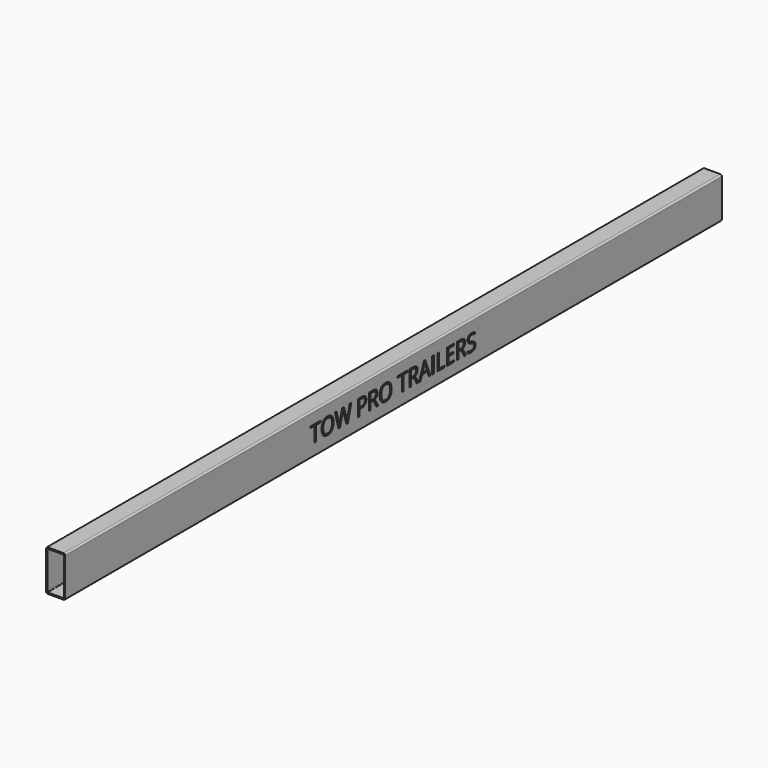
from build123d import *

# Parameters (mm, degrees)
F1_DEPTH      = 1500
F2_TEXT_SIZE  = 41.6666666667
F3_DEPTH      = 25
F3_DEPTH_BACK = 25


# Not quite as in the source:
# - Text() gives the source's letters only with a copy of the font that has no kerning and outlines rounded to 1/6400 em; it was checked with that copy


with BuildPart() as f1:
    # F0 (on Front) → F1 (new body)
    with BuildSketch(Plane.XZ):
        with BuildLine():
            ThreePointArc((17.5, 34.5), (16.6213203436, 36.6213203436), (14.5, 37.5))
            Line((14.5, 37.5), (-14.5, 37.5))
            ThreePointArc((-14.5, 37.5), (-16.6213203436, 36.6213203436), (-17.5, 34.5))
            Line((-17.5, 34.5), (-17.5, -34.5))
            ThreePointArc((-17.5, -34.5), (-16.6213203436, -36.6213203436), (-14.5, -37.5))
            Line((-14.5, -37.5), (14.5, -37.5))
            ThreePointArc((14.5, -37.5), (16.6213203436, -36.6213203436), (17.5, -34.5))
            Line((17.5, -34.5), (17.5, 34.5))
        make_face()
        with BuildLine():
            ThreePointArc((14, 35), (14.7071067812, 34.7071067812), (15, 34))
            Line((15, 34), (15, -34))
            ThreePointArc((15, -34), (14.7071067812, -34.7071067812), (14, -35))
            Line((14, -35), (-14, -35))
            ThreePointArc((-14, -35), (-14.7071067812, -34.7071067812), (-15, -34))
            Line((-15, -34), (-15, 34))
            ThreePointArc((-15, 34), (-14.7071067812, 34.7071067812), (-14, 35))
            Line((-14, 35), (14, 35))
        make_face(mode=Mode.SUBTRACT)
    extrude(amount=-F1_DEPTH)

    # F2 (on face) → F3 (cut, two sides)
    with BuildSketch(Plane.YZ.offset(17.5)) as f3_sk:
        with Locations((560.0325520833, -15)):
            Text('TOW PRO TRAILERS', F2_TEXT_SIZE, font='Open Sans', text_align=(TextAlign.LEFT, TextAlign.BOTTOM))
    extrude(amount=F3_DEPTH, mode=Mode.SUBTRACT)
    extrude(f3_sk.sketch, amount=-F3_DEPTH_BACK, mode=Mode.SUBTRACT)


solid = f1.part
